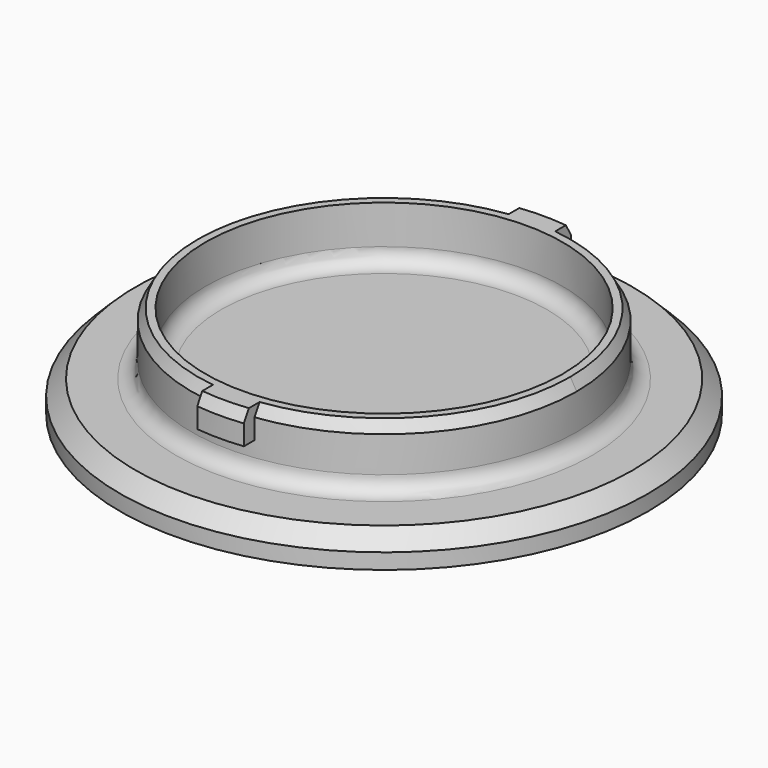
from build123d import *

# Parameters (mm, degrees)
F0_R          = 17
F1_DEPTH      = 2
F2_R          = 12.4
F3_DEPTH      = 4
F4_R          = 11.5
F5_DEPTH      = 3.5
F7_DEPTH      = 2
F8_R          = 1
F9_SIZE       = 1
F10_T4_ANGLE  = 182.8625440008
F10_T9_ANGLE  = 91.4226768156
F10_T12_ANGLE = 28.6625731368
F10_T14_ANGLE = 28.6625731368
F10_T18_ANGLE = 91.4226768156


# Not quite as in the source:
# - a fillet or chamfer that OpenCascade refuses, or shapes differently, is made with other operations: its cross-section is extruded or revolved along the edge and cut away or added


with BuildPart() as f1:
    # F0 (on Top) → F1 (new body)
    with BuildSketch(Plane.XY):
        Circle(F0_R)
    extrude(amount=F1_DEPTH)

    # F2 (on face) → F3 (join)
    with BuildSketch(Plane.XY.offset(2)):
        Circle(F2_R)
    extrude(amount=F3_DEPTH)

    # F4 (on face) → F5 (cut)
    with BuildSketch(Plane.XY.offset(6)):
        Circle(F4_R)
    extrude(amount=-F5_DEPTH, mode=Mode.SUBTRACT)

    # F6 (on face) → F7 (join)
    with BuildSketch(Plane.XY.offset(6)):
        with BuildLine():
            Line((-1.5, 13.1648205457), (-1.5, 12.3089398406))
            ThreePointArc((-1.5, 12.3089398406), (0, 12.4), (1.5, 12.3089398406))
            Line((1.5, 12.3089398406), (1.5, 13.1648205457))
            ThreePointArc((1.5, 13.1648205457), (0, 13.25), (-1.5, 13.1648205457))
        make_face()
        with BuildLine():
            Line((-1.5, -12.3089398406), (-1.5, -13.1648205457))
            ThreePointArc((-1.5, -13.1648205457), (0, -13.25), (1.5, -13.1648205457))
            Line((1.5, -13.1648205457), (1.5, -12.3089398406))
            ThreePointArc((1.5, -12.3089398406), (0, -12.4), (-1.5, -12.3089398406))
        make_face()
    extrude(amount=-F7_DEPTH)

    # F8
    f8_edges = [f1.edges().sort_by_distance(p)[0] for p in [
        (-11.5, 0, 2.5),
        (-12.4, 0, 2),
    ]]
    fillet(f8_edges, radius=F8_R)

    # F9
    f9_edges = [f1.edges().sort_by_distance(p)[0] for p in [
        (-17, 0, 2),
    ]]
    chamfer(f9_edges, length=F9_SIZE)

    # F10: chamfer of 0.7 x 0.4041451884 on 5 edges, made by hand


with BuildPart() as f10_tool2:
    # F10_s3 → F10_t4 (revolve)
    with BuildSketch(Plane(origin=(0, 0, 0), x_dir=(0, 0, 1), z_dir=(0.9996880058, -0.0249778109, 0))):
        Polygon((5.3, -12.4), (6, -11.9958548116), (6, -12.4), align=None)
    revolve(axis=Axis((0, 0, 6), (0, 0, 1)), revolution_arc=F10_T4_ANGLE)

    split(bisect_by=Plane.YZ.offset(-1.5), keep=Keep.BOTTOM)


with BuildPart() as f1_1:
    add(f1.part)

    # F10_t1: cut F10_tool2
    add(f10_tool2.part, mode=Mode.SUBTRACT)


with BuildPart() as f10_tool7:
    # F10_s8 → F10_t9 (revolve)
    with BuildSketch(Plane.XZ):
        Polygon((12.4, 5.3), (11.9958548116, 6), (12.4, 6), align=None)
    revolve(axis=Axis((0, 0, 6), (0, 0, 1)), revolution_arc=F10_T9_ANGLE)

    split(bisect_by=Plane.YZ.offset(1.5), keep=Keep.TOP)


with BuildPart() as f1_2:
    add(f1_1.part)

    # F10_t6: cut F10_tool7
    add(f10_tool7.part, mode=Mode.SUBTRACT)

    # F10_s11 → F10_t12 (revolve, cut)
    with BuildSketch(Plane(origin=(0, 0, 0), x_dir=(0, 0, 1), z_dir=(-0.9688807122, 0.2475281104, 0))):
        Polygon((6, -12.8458548116), (5.3, -13.25), (6, -13.25), align=None)
    revolve(axis=Axis((0, 0, 6), (0, 0, 1)), revolution_arc=F10_T12_ANGLE, mode=Mode.SUBTRACT)

    # F10_s13 → F10_t14 (revolve, cut)
    with BuildSketch(Plane(origin=(0, 0, 0), x_dir=(0, 0, 1), z_dir=(0.9688807122, -0.2475281104, 0))):
        Polygon((6, -12.8458548116), (5.3, -13.25), (6, -13.25), align=None)
    revolve(axis=Axis((0, 0, 6), (0, 0, 1)), revolution_arc=F10_T14_ANGLE, mode=Mode.SUBTRACT)


with BuildPart() as f10_tool16:
    # F10_s17 → F10_t18 (revolve)
    with BuildSketch(Plane(origin=(0, 0, 0), x_dir=(0, 0, 1), z_dir=(-0.9996917416, 0.0248278432, 0))):
        Polygon((5.3, -12.4), (6, -11.9958548116), (6, -12.4), align=None)
    revolve(axis=Axis((0, 0, 6), (0, 0, 1)), revolution_arc=F10_T18_ANGLE)

    split(bisect_by=Plane.YZ.offset(1.5), keep=Keep.TOP)


with BuildPart() as f1_3:
    add(f1_2.part)

    # F10_t15: cut F10_tool16
    add(f10_tool16.part, mode=Mode.SUBTRACT)


with BuildPart() as f11_1:
    # F11: copy of F1
    add(f1_3.part)


solid = Compound([f1_3.part, f11_1.part])
